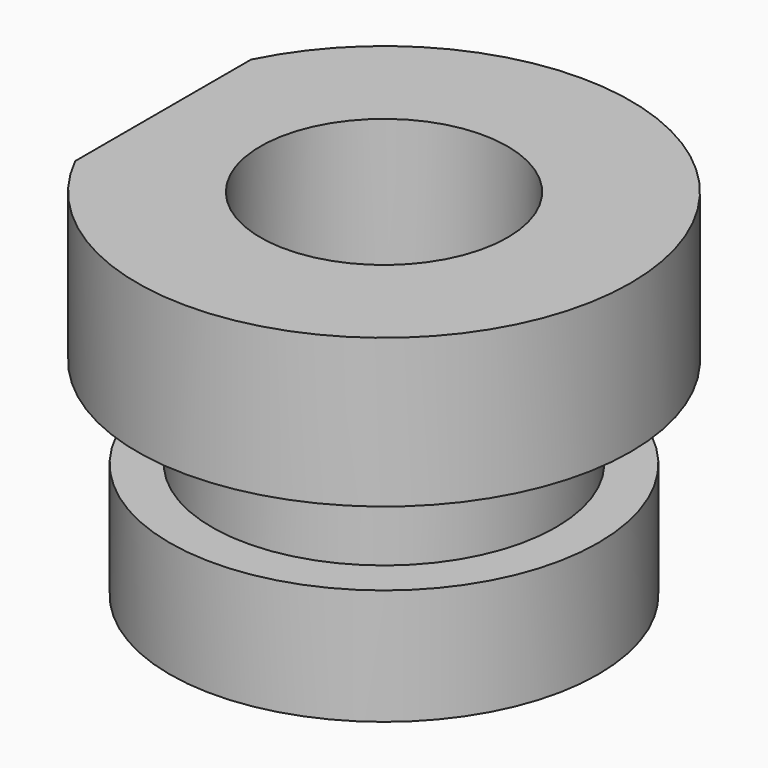
from build123d import *

# Parameters (mm, degrees)
F0_R     = 11
F0_R_2   = 7.9
F1_DEPTH = 9.5
F2_DEPTH = 5.8
F3_R     = 13.7
F3_R_2   = 11
F3_R_3   = 7.9
F4_DEPTH = 7.4


with BuildPart() as f1:
    # F0 (on Top) → F1 (new body)
    with BuildSketch(Plane.XY):
        with BuildLine():
            Line((-14.125, 7.0238878123), (-14.125, -7.0238878123))
            ThreePointArc((-14.125, -7.0238878123), (15.775, 0), (-14.125, 7.0238878123))
        make_face()
        Circle(F0_R, mode=Mode.SUBTRACT)
        Circle(F0_R)
        Circle(F0_R_2, mode=Mode.SUBTRACT)
    extrude(amount=F1_DEPTH)

    # F0 (on Top) → F2 (join)
    with BuildSketch(Plane.XY):
        Circle(F0_R)
        Circle(F0_R_2, mode=Mode.SUBTRACT)
    extrude(amount=-F2_DEPTH)

    # F3 (on face) → F4 (join)
    with BuildSketch(Plane(origin=(0, 0, -5.8), x_dir=(1, 0, 0), z_dir=(0, 0, -1))):
        Circle(F3_R)
        Circle(F3_R_2, mode=Mode.SUBTRACT)
        Circle(F3_R_2)
        Circle(F3_R_3, mode=Mode.SUBTRACT)
    extrude(amount=F4_DEPTH)


solid = f1.part
